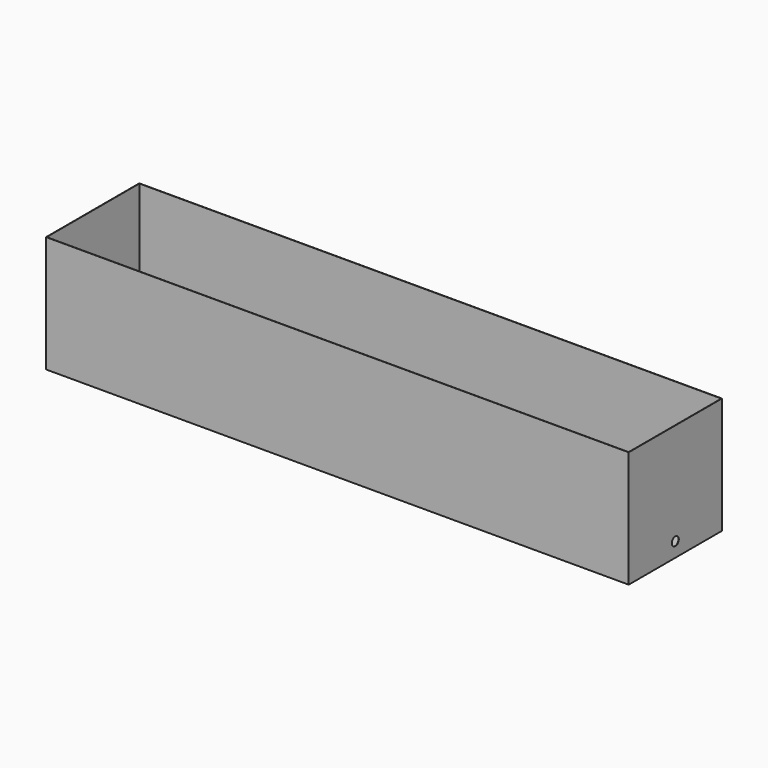
from build123d import *

# Parameters (mm, degrees)
F0_W     = 2000
F0_H     = 400
F1_DEPTH = 400
F2_T     = -1
F5_D     = 40
F8_D     = 30


# Not quite as in the source:
# - the program builds the solid bodies; features that only make, move or delete a surface that nothing else refers to are left out


with BuildPart() as f1:
    # F0 (on Top) → F1 (new body)
    with BuildSketch(Plane.XY):
        Rectangle(F0_W, F0_H)
    extrude(amount=F1_DEPTH)

    # F2
    f2_openings = [f1.faces().sort_by_distance(p)[0] for p in [
        (0, 0, 400),
    ]]
    offset(amount=F2_T, openings=f2_openings)

    # F5 (through all)
    with Locations(Plane.XY.offset(1)):
        with Locations((977, 177), (977, -177), (-977, 177), (-977, -177)):
            Hole(F5_D / 2)

    # F8 (through all)
    with Locations(Plane(origin=(-1000, 0, 0), x_dir=(0, -1, 0), z_dir=(-1, 0, 0))):
        with Locations((0, 50)):
            Hole(F8_D / 2)


solid = f1.part
